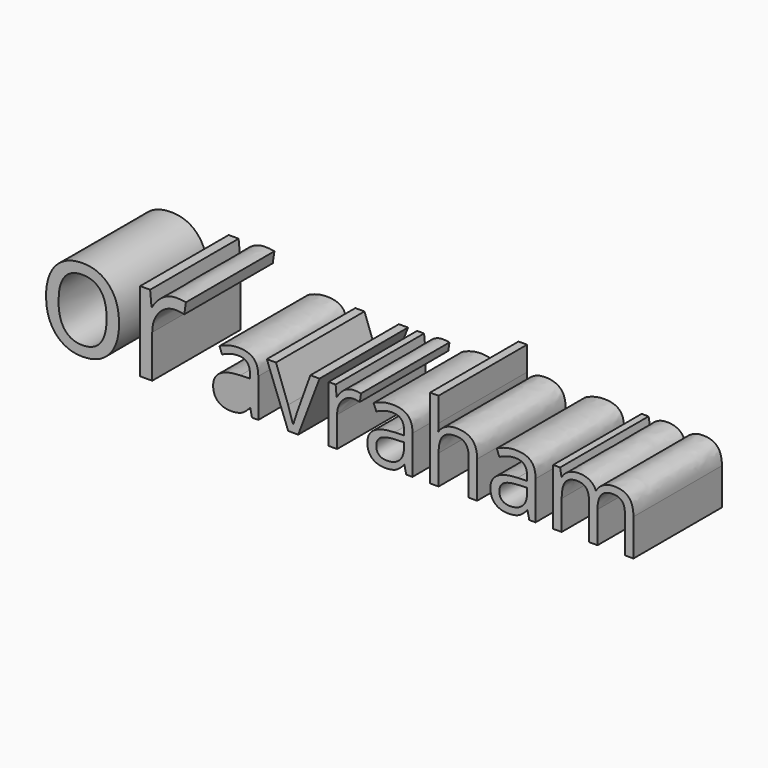
from build123d import *

# Parameters (mm, degrees)
F0_TEXT_SIZE = 34.0949200715
F1_DEPTH     = 25.4
F2_TEXT_SIZE = 24.1615085138
F3_DEPTH     = 25.4


# Not quite as in the source:
# - Text() gives the source's letters only with a copy of the font that has no kerning and outlines rounded to 1/6400 em; it was checked with that copy


with BuildPart() as f1:
    # F0 (on Front) → F1 (new body)
    with BuildSketch(Plane.XZ):
        with Locations((-153.7946611643, 31.5990778618)):
            Text('or', F0_TEXT_SIZE, font='Open Sans', text_align=(TextAlign.LEFT, TextAlign.BOTTOM))
    extrude(amount=F1_DEPTH)


with BuildPart() as f3:
    # F2 (on Front) → F3 (new body)
    with BuildSketch(Plane.XZ):
        with Locations((-114.6230697632, 31.6027067602)):
            Text('avraham', F2_TEXT_SIZE, font='Open Sans', text_align=(TextAlign.LEFT, TextAlign.BOTTOM))
        with BuildLine():
            add(Edge.make_bspline(
                [(-110.8176321723, 33.5375150591), (-110.1758421024, 32.9844430283), (-109.0206199765, 32.9844430283)],
                knots=[0, 0, 0, 1, 1, 1], degree=2))
            add(Edge.make_bspline(
                [(-109.0206199765, 32.9844430283), (-107.1896306595, 32.9844430283), (-106.145777987, 33.9867681081)],
                knots=[0, 0, 0, 1, 1, 1], degree=2))
            add(Edge.make_bspline(
                [(-106.145777987, 33.9867681081), (-105.1019253145, 34.9890931878), (-105.1019253145, 36.7936558549)],
                knots=[0, 0, 0, 1, 1, 1], degree=2))
            Line((-105.1019253145, 36.7936558549), (-105.1019253145, 37.9602036879))
            Line((-105.1019253145, 37.9602036879), (-107.0612726455, 37.8809237381))
            add(Edge.make_bspline(
                [(-107.0612726455, 37.8809237381), (-109.3981435471, 37.7978685525), (-110.4287828946, 37.1541908648)],
                knots=[0, 0, 0, 1, 1, 1], degree=2))
            add(Edge.make_bspline(
                [(-110.4287828946, 37.1541908648), (-111.4594222422, 36.510513177), (-111.4594222422, 35.1552035588)],
                knots=[0, 0, 0, 1, 1, 1], degree=2))
            add(Edge.make_bspline(
                [(-111.4594222422, 35.1552035588), (-111.4594222422, 34.09058709), (-110.8176321723, 33.5375150591)],
                knots=[0, 0, 0, 1, 1, 1], degree=2))
        make_face()
    extrude(amount=F3_DEPTH)


solid = Compound([f1.part, f3.part])
